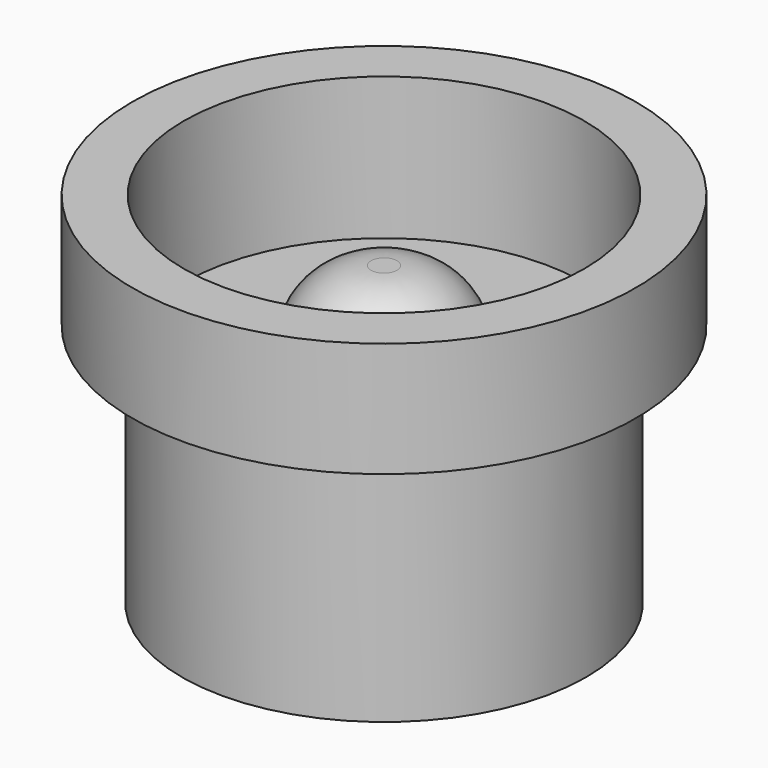
from build123d import *

# Parameters (mm, degrees)
F2_R     = 8.5041977155
F3_DEPTH = 6.0452
F4_R     = 3.5986110649
F5_DEPTH = 3.4036
F6_R     = 3.048


# Not quite as in the source:
# - a feature of the source that left no trace in its solid (it failed there, or was rolled back) is left out


with BuildPart() as f1:
    # F0 (on Front) → F1 (revolve)
    with BuildSketch(Plane.XZ):
        Polygon((0, -7.3331215731), (0, 7.9068784269), (-10.6934, 7.9068784269), (-10.6934, 3.0300784269), (-8.5852, 3.0300784269), (-8.5852, -7.3331215731), align=None)
    revolve(axis=Axis((0, 0, 0.2868784269), (0, 0, 1)))

    # F2 (on face) → F3 (cut)
    with BuildSketch(Plane.XY.offset(7.9068784269)):
        Circle(F2_R)
    extrude(amount=-F3_DEPTH, mode=Mode.SUBTRACT)

    # F4 (on face) → F5 (join)
    with BuildSketch(Plane.XY.offset(1.8616784269)):
        Circle(F4_R)
    extrude(amount=F5_DEPTH)

    # F6
    f6_edges = [f1.edges().sort_by_distance(p)[0] for p in [
        (-3.598611, 0, 5.265278),
    ]]
    fillet(f6_edges, radius=F6_R)


solid = f1.part
